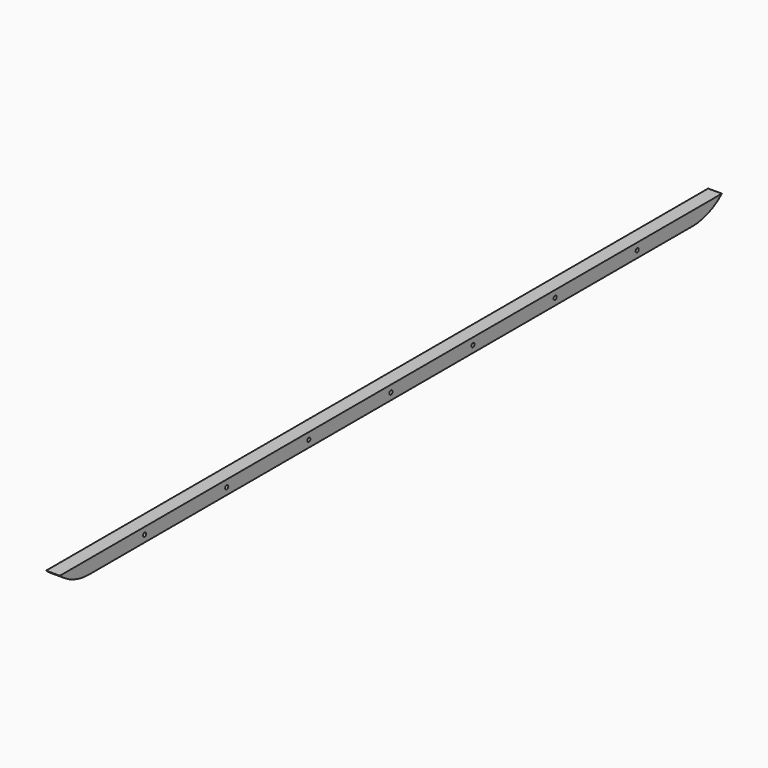
from build123d import *

# Parameters (mm, degrees)
F0_W        = 6.35
F0_H        = 6.35
F1_DEPTH    = 190.5
F2_T1_DEPTH = 90.3526041263
F4_D        = 1.778


# Not quite as in the source:
# - a fillet or chamfer that OpenCascade refuses, or shapes differently, is made with other operations: its cross-section is extruded or revolved along the edge and cut away or added


with BuildPart() as f1:
    # F0 (on Front) → F1 (new body, symmetric)
    with BuildSketch(Plane.XZ):
        Rectangle(F0_W, F0_H)
    extrude(amount=F1_DEPTH, both=True)

    # F2: fillet of radius 25.4 on 2 edges, made by hand

    # F2_s2 → F2_t1 (cut)
    with BuildSketch(Plane.YZ.offset(-45.1763020632)):
        with BuildLine():
            ThreePointArc((-173.6994791747, -3.175), (-182.6797352958, -1.534524406), (-190.5, 3.175))
            Line((-190.5, 3.175), (-190.5, -3.175))
            Line((-190.5, -3.175), (-173.6994791747, -3.175))
        make_face()
        with BuildLine():
            ThreePointArc((173.6994791747, -3.175), (182.6797352958, -1.534524406), (190.5, 3.175))
            Line((190.5, 3.175), (190.5, -3.175))
            Line((190.5, -3.175), (173.6994791747, -3.175))
        make_face()
    extrude(amount=F2_T1_DEPTH, mode=Mode.SUBTRACT)

    # F4 (through all)
    with Locations(Plane.YZ.offset(3.175)):
        with Locations((47.244, 0), (94.488, 0), (141.732, 0), (0, 0), (-47.244, 0), (-94.488, 0), (-141.732, 0)):
            Hole(F4_D / 2)


solid = f1.part
